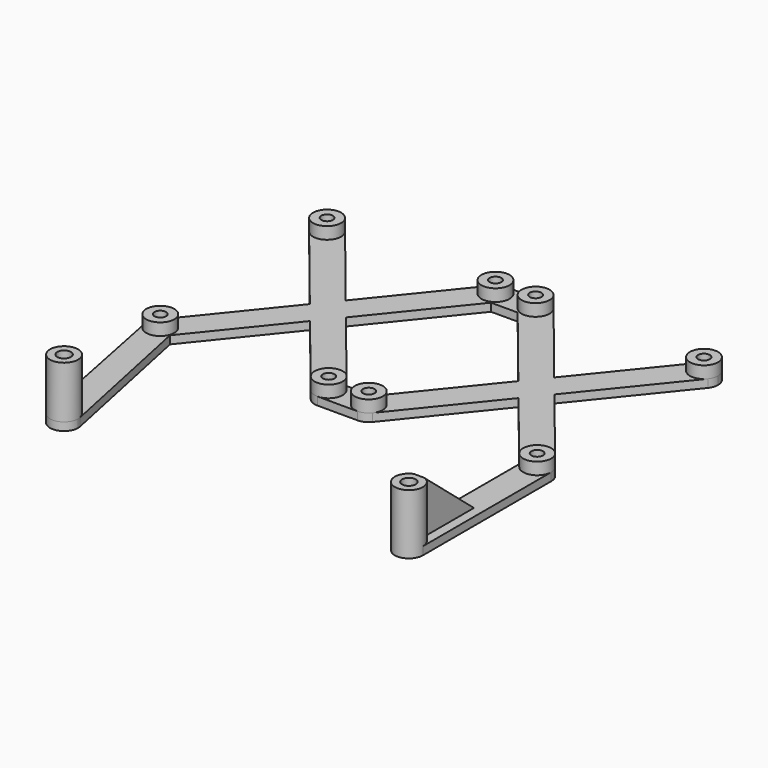
from build123d import *

# Parameters (mm, degrees)
F0_R        = 1.45
F0_R_2      = 1.7
F1_DEPTH    = 2
F2_R        = 3.5
F2_R_2      = 1.45
F3_DEPTH    = 3
F4_R        = 3.5
F4_R_2      = 1.7
F5_DEPTH    = 13
F6_W        = 2.2071525455
F6_H        = 17.9247483611
F7_DEPTH    = 13
F8_T4_DEPTH = 95.0013732124


# Not quite as in the source:
# - a fillet or chamfer that OpenCascade refuses, or shapes differently, is made with other operations: its cross-section is extruded or revolved along the edge and cut away or added


with BuildPart() as f1:
    # F0 (on Top) → F1 (new body)
    with BuildSketch(Plane.XY):
        with BuildLine():
            Line((21, -31.5702583224), (16.5009452012, -26))
            Line((16.5009452012, -26), (-2.7227941307, -49.8008201252))
            ThreePointArc((-2.7227941307, -49.8008201252), (0, -48.5), (2.7227941307, -49.8008201252))
            ThreePointArc((2.7227941307, -49.8008201252), (3.2999832922, -50.8337623436), (3.5, -52))
            ThreePointArc((3.5, -52), (3.4691335198, -52.4638023524), (3.3770785016, -52.9194241642))
            Line((3.3770785016, -52.9194241642), (3.4553009961, -53.2922666129))
            Line((3.4553009961, -53.2922666129), (21, -31.5702583224))
        make_face()
        with BuildLine():
            ThreePointArc((2.7227941307, 2.1991798748), (3.2999832922, 1.1662376564), (3.5, 0))
            ThreePointArc((3.5, 0), (1.1662376564, -3.2999832922), (-2.7227941307, -2.1991798748))
            Line((-2.7227941307, -2.1991798748), (16.5009452012, -26))
            Line((16.5009452012, -26), (21, -20.4297416776))
            Line((21, -20.4297416776), (2.7227941307, 2.1991798748))
        make_face()
        with BuildLine():
            Line((39.2772058693, 2.1991798748), (21, -20.4297416776))
            Line((21, -20.4297416776), (25.4990547988, -26))
            Line((25.4990547988, -26), (43.6721317219, -3.5))
            Line((43.6721317219, -3.5), (42, -3.5))
            ThreePointArc((42, -3.5), (38.841904881, -1.5087860084), (39.2772058693, 2.1991798748))
        make_face()
        Polygon((25.4990547988, -26), (21, -20.4297416776), (16.5009452012, -26), (21, -31.5702583224), align=None)
        with BuildLine():
            Line((43.6721317219, -48.5), (25.4990547988, -26))
            Line((25.4990547988, -26), (21, -31.5702583224))
            Line((21, -31.5702583224), (39.2772058693, -54.1991798748))
            ThreePointArc((39.2772058693, -54.1991798748), (38.841904881, -50.4912139916), (42, -48.5))
            Line((42, -48.5), (43.6721317219, -48.5))
        make_face()
        with BuildLine():
            Line((50.3278682781, -48.5), (43.6721317219, -48.5))
            Line((43.6721317219, -48.5), (44.7227941307, -49.8008201252))
            ThreePointArc((44.7227941307, -49.8008201252), (45.2999832922, -50.8337623436), (45.5, -52))
            ThreePointArc((45.5, -52), (44.4748737342, -54.4748737342), (42, -55.5))
            Line((42, -55.5), (52, -55.5))
            ThreePointArc((52, -55.5), (48.841904881, -53.5087860084), (49.2772058693, -49.8008201252))
            Line((49.2772058693, -49.8008201252), (50.3278682781, -48.5))
        make_face()
        with BuildLine():
            Line((11.425424692, -91.2813445337), (3.4553009961, -53.2922666129))
            Line((3.4553009961, -53.2922666129), (2.7227941307, -54.1991798748))
            ThreePointArc((2.7227941307, -54.1991798748), (-0.8353894658, -55.3988416322), (-3.4320323649, -52.686406473))
            Line((-3.4320323649, -52.686406473), (4.5679676351, -92.686406473))
            ThreePointArc((4.5679676351, -92.686406473), (7.2974612618, -88.5712335569), (11.425424692, -91.2813445337))
        make_face()
        with BuildLine():
            Line((68.5009452012, -26), (50.3278682781, -48.5))
            Line((50.3278682781, -48.5), (52, -48.5))
            ThreePointArc((52, -48.5), (54.4748737342, -49.5251262658), (55.5, -52))
            ThreePointArc((55.5, -52), (55.2999832922, -53.1662376564), (54.7227941307, -54.1991798748))
            Line((54.7227941307, -54.1991798748), (73, -31.5702583224))
            Line((73, -31.5702583224), (68.5009452012, -26))
        make_face()
        with BuildLine():
            Line((52, -3.5), (50.3278682781, -3.5))
            Line((50.3278682781, -3.5), (68.5009452012, -26))
            Line((68.5009452012, -26), (73, -20.4297416776))
            Line((73, -20.4297416776), (54.7227941307, 2.1991798748))
            ThreePointArc((54.7227941307, 2.1991798748), (55.2999832922, 1.1662376564), (55.5, 0))
            ThreePointArc((55.5, 0), (54.4748737342, -2.4748737342), (52, -3.5))
        make_face()
        with BuildLine():
            Line((44.7227941307, -2.1991798748), (43.6721317219, -3.5))
            Line((43.6721317219, -3.5), (50.3278682781, -3.5))
            Line((50.3278682781, -3.5), (49.2772058693, -2.1991798748))
            ThreePointArc((49.2772058693, -2.1991798748), (48.841904881, 1.5087860084), (52, 3.5))
            Line((52, 3.5), (42, 3.5))
            ThreePointArc((42, 3.5), (44.4748737342, 2.4748737342), (45.5, 0))
            ThreePointArc((45.5, 0), (45.2999832922, -1.1662376564), (44.7227941307, -2.1991798748))
        make_face()
        Polygon((73, -20.4297416776), (68.5009452012, -26), (73, -31.5702583224), (77.4990547988, -26), align=None)
        with BuildLine():
            Line((91.2772058693, 2.1991798748), (73, -20.4297416776))
            Line((73, -20.4297416776), (77.4990547988, -26))
            Line((77.4990547988, -26), (96.7227941307, -2.1991798748))
            ThreePointArc((96.7227941307, -2.1991798748), (91.8008201252, -2.7227941307), (91.2772058693, 2.1991798748))
        make_face()
        with BuildLine():
            Line((77.4990547988, -26), (73, -31.5702583224))
            Line((73, -31.5702583224), (90.5, -53.236924989))
            Line((90.5, -53.236924989), (90.5, -52))
            ThreePointArc((90.5, -52), (92.8337623436, -48.7000167078), (96.7227941307, -49.8008201252))
            Line((96.7227941307, -49.8008201252), (77.4990547988, -26))
        make_face()
        with BuildLine():
            Line((91.2772058693, -54.1991798748), (90.5, -53.236924989))
            Line((90.5, -53.236924989), (90.5, -92))
            ThreePointArc((90.5, -92), (94, -88.5), (97.5, -92))
            Line((97.5, -92), (97.5, -52))
            ThreePointArc((97.5, -52), (95.1662376564, -55.2999832922), (91.2772058693, -54.1991798748))
        make_face()
        with BuildLine():
            ThreePointArc((-2.7227941307, -2.1991798748), (1.1662376564, -3.2999832922), (3.5, 0))
            ThreePointArc((3.5, 0), (3.2999832922, 1.1662376564), (2.7227941307, 2.1991798748))
            ThreePointArc((2.7227941307, 2.1991798748), (-2.1991798748, 2.7227941307), (-2.7227941307, -2.1991798748))
        make_face()
        Circle(F0_R, mode=Mode.SUBTRACT)
        with BuildLine():
            ThreePointArc((42, 3.5), (40.4912139916, 3.158095119), (39.2772058693, 2.1991798748))
            ThreePointArc((39.2772058693, 2.1991798748), (38.841904881, -1.5087860084), (42, -3.5))
            ThreePointArc((42, -3.5), (43.5087860084, -3.158095119), (44.7227941307, -2.1991798748))
            ThreePointArc((44.7227941307, -2.1991798748), (45.2999832922, -1.1662376564), (45.5, 0))
            ThreePointArc((45.5, 0), (44.4748737342, 2.4748737342), (42, 3.5))
        make_face()
        with Locations((42, 0)):
            Circle(F0_R, mode=Mode.SUBTRACT)
        with BuildLine():
            ThreePointArc((54.7227941307, 2.1991798748), (53.5087860084, 3.158095119), (52, 3.5))
            ThreePointArc((52, 3.5), (48.841904881, 1.5087860084), (49.2772058693, -2.1991798748))
            ThreePointArc((49.2772058693, -2.1991798748), (50.4912139916, -3.158095119), (52, -3.5))
            ThreePointArc((52, -3.5), (54.4748737342, -2.4748737342), (55.5, 0))
            ThreePointArc((55.5, 0), (55.2999832922, 1.1662376564), (54.7227941307, 2.1991798748))
        make_face()
        with Locations((52, 0)):
            Circle(F0_R, mode=Mode.SUBTRACT)
        with BuildLine():
            ThreePointArc((97.5, 0), (95.1662376564, 3.2999832922), (91.2772058693, 2.1991798748))
            ThreePointArc((91.2772058693, 2.1991798748), (91.8008201252, -2.7227941307), (96.7227941307, -2.1991798748))
            ThreePointArc((96.7227941307, -2.1991798748), (97.2999832922, -1.1662376564), (97.5, 0))
        make_face()
        with Locations((94, 0)):
            Circle(F0_R, mode=Mode.SUBTRACT)
        with BuildLine():
            ThreePointArc((97.5, -52), (97.2999832922, -50.8337623436), (96.7227941307, -49.8008201252))
            ThreePointArc((96.7227941307, -49.8008201252), (92.8337623436, -48.7000167078), (90.5, -52))
            ThreePointArc((90.5, -52), (90.7000167078, -53.1662376564), (91.2772058693, -54.1991798748))
            ThreePointArc((91.2772058693, -54.1991798748), (95.1662376564, -55.2999832922), (97.5, -52))
        make_face()
        with Locations((94, -52)):
            Circle(F0_R, mode=Mode.SUBTRACT)
        with BuildLine():
            ThreePointArc((97.5, -92), (94, -88.5), (90.5, -92))
            ThreePointArc((90.5, -92), (94, -95.5), (97.5, -92))
        make_face()
        with Locations((94, -92)):
            Circle(F0_R_2, mode=Mode.SUBTRACT)
        with BuildLine():
            ThreePointArc((52, -48.5), (50.4912139916, -48.841904881), (49.2772058693, -49.8008201252))
            ThreePointArc((49.2772058693, -49.8008201252), (48.841904881, -53.5087860084), (52, -55.5))
            ThreePointArc((52, -55.5), (53.5087860084, -55.158095119), (54.7227941307, -54.1991798748))
            ThreePointArc((54.7227941307, -54.1991798748), (55.2999832922, -53.1662376564), (55.5, -52))
            ThreePointArc((55.5, -52), (54.4748737342, -49.5251262658), (52, -48.5))
        make_face()
        with Locations((52, -52)):
            Circle(F0_R, mode=Mode.SUBTRACT)
        with BuildLine():
            ThreePointArc((42, -48.5), (38.841904881, -50.4912139916), (39.2772058693, -54.1991798748))
            ThreePointArc((39.2772058693, -54.1991798748), (40.4912139916, -55.158095119), (42, -55.5))
            ThreePointArc((42, -55.5), (44.4748737342, -54.4748737342), (45.5, -52))
            ThreePointArc((45.5, -52), (45.2999832922, -50.8337623436), (44.7227941307, -49.8008201252))
            ThreePointArc((44.7227941307, -49.8008201252), (43.5087860084, -48.841904881), (42, -48.5))
        make_face()
        with Locations((42, -52)):
            Circle(F0_R, mode=Mode.SUBTRACT)
        with BuildLine():
            ThreePointArc((11.5, -92), (11.4813062507, -91.6387427662), (11.425424692, -91.2813445337))
            ThreePointArc((11.425424692, -91.2813445337), (7.2974612618, -88.5712335569), (4.5679676351, -92.686406473))
            ThreePointArc((4.5679676351, -92.686406473), (8.3448816629, -95.4829666433), (11.5, -92))
        make_face()
        with Locations((8, -92)):
            Circle(F0_R_2, mode=Mode.SUBTRACT)
        with BuildLine():
            Line((2.7227941307, -54.1991798748), (3.4553009961, -53.2922666129))
            Line((3.4553009961, -53.2922666129), (3.3770785016, -52.9194241642))
            ThreePointArc((3.3770785016, -52.9194241642), (3.1163368243, -53.5932497599), (2.7227941307, -54.1991798748))
        make_face()
        with BuildLine():
            ThreePointArc((3.5, -52), (3.2999832922, -50.8337623436), (2.7227941307, -49.8008201252))
            Line((2.7227941307, -49.8008201252), (3.3770785016, -52.9194241642))
            ThreePointArc((3.3770785016, -52.9194241642), (3.4691335198, -52.4638023524), (3.5, -52))
        make_face()
        with BuildLine():
            ThreePointArc((2.7227941307, -49.8008201252), (0, -48.5), (-2.7227941307, -49.8008201252))
            ThreePointArc((-2.7227941307, -49.8008201252), (-3.3988416322, -51.1646105342), (-3.4320323649, -52.686406473))
            ThreePointArc((-3.4320323649, -52.686406473), (-0.8353894658, -55.3988416322), (2.7227941307, -54.1991798748))
            ThreePointArc((2.7227941307, -54.1991798748), (3.1163368243, -53.5932497599), (3.3770785016, -52.9194241642))
            Line((3.3770785016, -52.9194241642), (2.7227941307, -49.8008201252))
        make_face()
        with Locations((0, -52)):
            Circle(F0_R, mode=Mode.SUBTRACT)
        with BuildLine():
            Line((44.7227941307, -49.8008201252), (43.6721317219, -48.5))
            Line((43.6721317219, -48.5), (42, -48.5))
            ThreePointArc((42, -48.5), (43.5087860084, -48.841904881), (44.7227941307, -49.8008201252))
        make_face()
        with BuildLine():
            Line((52, -48.5), (50.3278682781, -48.5))
            Line((50.3278682781, -48.5), (49.2772058693, -49.8008201252))
            ThreePointArc((49.2772058693, -49.8008201252), (50.4912139916, -48.841904881), (52, -48.5))
        make_face()
        with BuildLine():
            Line((42, -3.5), (43.6721317219, -3.5))
            Line((43.6721317219, -3.5), (44.7227941307, -2.1991798748))
            ThreePointArc((44.7227941307, -2.1991798748), (43.5087860084, -3.158095119), (42, -3.5))
        make_face()
        with BuildLine():
            Line((49.2772058693, -2.1991798748), (50.3278682781, -3.5))
            Line((50.3278682781, -3.5), (52, -3.5))
            ThreePointArc((52, -3.5), (50.4912139916, -3.158095119), (49.2772058693, -2.1991798748))
        make_face()
        with BuildLine():
            Line((90.5, -52), (90.5, -53.236924989))
            Line((90.5, -53.236924989), (91.2772058693, -54.1991798748))
            ThreePointArc((91.2772058693, -54.1991798748), (90.7000167078, -53.1662376564), (90.5, -52))
        make_face()
    extrude(amount=F1_DEPTH)

    # F2 (on face) → F3 (join)
    with BuildSketch(Plane.XY.offset(2)):
        Circle(F2_R)
        Circle(F2_R_2, mode=Mode.SUBTRACT)
        with Locations((42, 0)):
            Circle(F2_R)
        with Locations((42, 0)):
            Circle(F2_R_2, mode=Mode.SUBTRACT)
        with Locations((42, -52)):
            Circle(F2_R)
        with Locations((42, -52)):
            Circle(F2_R_2, mode=Mode.SUBTRACT)
        with Locations((0, -52)):
            Circle(F2_R)
        with Locations((0, -52)):
            Circle(F2_R_2, mode=Mode.SUBTRACT)
        with Locations((52, 0)):
            Circle(F2_R)
        with Locations((52, 0)):
            Circle(F2_R_2, mode=Mode.SUBTRACT)
        with Locations((94, 0)):
            Circle(F2_R)
        with Locations((94, 0)):
            Circle(F2_R_2, mode=Mode.SUBTRACT)
        with Locations((94, -52)):
            Circle(F2_R)
        with Locations((94, -52)):
            Circle(F2_R_2, mode=Mode.SUBTRACT)
        with Locations((52, -52)):
            Circle(F2_R)
        with Locations((52, -52)):
            Circle(F2_R_2, mode=Mode.SUBTRACT)
    extrude(amount=F3_DEPTH)

    # F4 (on face) → F5 (join)
    with BuildSketch(Plane.XY.offset(2)):
        with Locations((8, -92)):
            Circle(F4_R)
        with Locations((8, -92)):
            Circle(F4_R_2, mode=Mode.SUBTRACT)
        with Locations((94, -92)):
            Circle(F4_R)
        with Locations((94, -92)):
            Circle(F4_R_2, mode=Mode.SUBTRACT)
    extrude(amount=F5_DEPTH)

    # F6 (on face) → F7 (join)
    with BuildSketch(Plane.XY.offset(2)):
        with Locations((94.0635614097, -79.7419138253)):
            Rectangle(F6_W, F6_H)
    extrude(amount=F7_DEPTH)

    # F8: chamfer of 15 x 18 on 1 edges, made by hand


with BuildPart() as f8_tool2:
    # F8_s3 → F8_t4 (new body)
    with BuildSketch(Plane.YZ.offset(141.5642480159)):
        Polygon((-88.7795396447, 15), (-70.7795396447, 0), (-70.7795396447, 15), align=None)
    extrude(amount=-F8_T4_DEPTH)

    split(bisect_by=Plane.XY.offset(2), keep=Keep.TOP)


with BuildPart() as f1_1:
    add(f1.part)

    # F8_t1: cut F8_tool2
    add(f8_tool2.part, mode=Mode.SUBTRACT)


solid = f1_1.part
